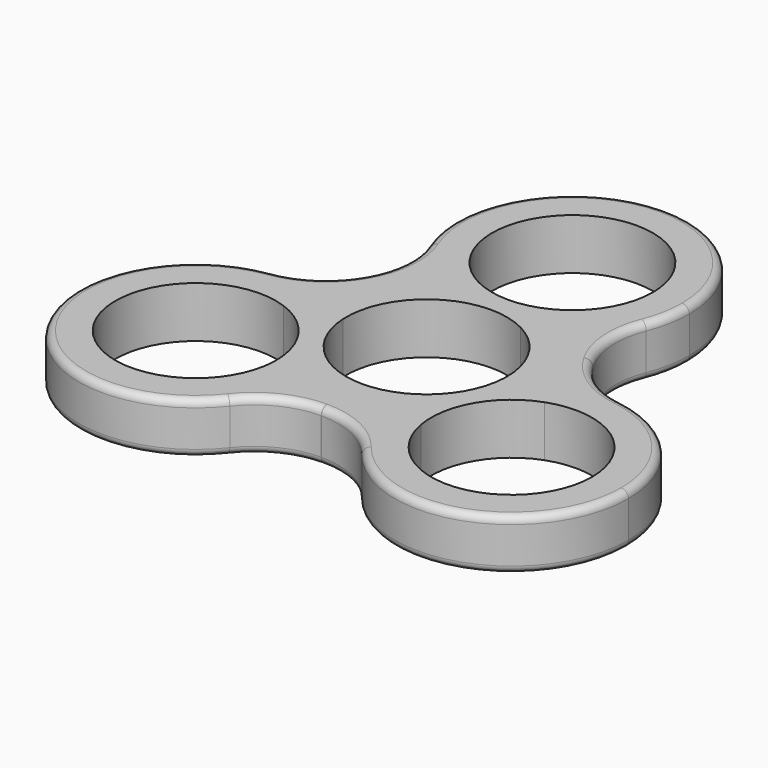
from build123d import *

# Parameters (mm, degrees)
F1_DEPTH = 7
F2_R     = 1


with BuildPart() as f1:
    # F0 (on Top) → F1 (new body)
    with BuildSketch(Plane.XY):
        with BuildLine():
            ThreePointArc((5.060494047, 9.795), (9.4165432051, 5.7340508426), (11.025, 0))
            ThreePointArc((11.025, 0), (11.0219910528, -0.2575620937), (11.0129658536, -0.5149835996))
            ThreePointArc((11.0129658536, -0.5149835996), (14.1740719643, 1.673977168), (17.7656075732, 3.0469349442))
            ThreePointArc((17.7656075732, 3.0469349442), (16.9557411525, 6.115837389), (15.6201357815, 8.9951088469))
            ThreePointArc((15.6201357815, 8.9951088469), (15.6101079032, 9.0125), (15.600060662, 9.0298799738))
            ThreePointArc((15.600060662, 9.0298799738), (13.7743411206, 11.6261838836), (11.5215268519, 13.862))
            ThreePointArc((11.5215268519, 13.862), (8.536742735, 11.4381178122), (5.060494047, 9.795))
        make_face()
        with BuildLine():
            ThreePointArc((-11.0129658536, -0.5149835996), (-9.5479300767, 5.5125), (-5.060494047, 9.795))
            ThreePointArc((-5.060494047, 9.795), (-8.536742735, 11.4381178122), (-11.5215268519, 13.862))
            ThreePointArc((-11.5215268519, 13.862), (-13.7743411206, 11.6261838836), (-15.600060662, 9.0298799738))
            ThreePointArc((-15.600060662, 9.0298799738), (-15.6101079032, 9.0125), (-15.6201357815, 8.9951088469))
            ThreePointArc((-15.6201357815, 8.9951088469), (-16.9557411525, 6.115837389), (-17.7656075732, 3.0469349442))
            ThreePointArc((-17.7656075732, 3.0469349442), (-14.1740719643, 1.673977168), (-11.0129658536, -0.5149835996))
        make_face()
        with BuildLine():
            ThreePointArc((7.1017699202, 16.567), (9.4093598037, 15.3741527599), (11.5215268519, 13.862))
            ThreePointArc((11.5215268519, 13.862), (13.4516295767, 16.2905633516), (14.8776527516, 19.0454997185))
            ThreePointArc((14.8776527516, 19.0454997185), (15.7355490903, 21.9679841973), (16.025, 25))
            ThreePointArc((16.025, 25), (-3.0320158027, 40.7355490903), (-14.8776527516, 19.0454997185))
            ThreePointArc((-14.8776527516, 19.0454997185), (-13.4516295767, 16.2905633516), (-11.5215268519, 13.862))
            ThreePointArc((-11.5215268519, 13.862), (-9.4093598037, 15.3741527599), (-7.1017699202, 16.567))
            ThreePointArc((-7.1017699202, 16.567), (-4.6504629678, 34.9961902335), (11.025, 25))
            ThreePointArc((11.025, 25), (9.9961902335, 20.3495370322), (7.1017699202, 16.567))
        make_face()
        with BuildLine():
            ThreePointArc((14.8776527516, 19.0454997185), (13.4516295767, 16.2905633516), (11.5215268519, 13.862))
            ThreePointArc((11.5215268519, 13.862), (13.7743411206, 11.6261838836), (15.600060662, 9.0298799738))
            ThreePointArc((15.600060662, 9.0298799738), (14.0855515443, 13.9545041029), (14.8776527516, 19.0454997185))
        make_face()
        with BuildLine():
            ThreePointArc((6.2440807213, -16.9089349442), (5.6373292293, -13.1120949802), (5.9524718066, -9.2800164004))
            ThreePointArc((5.9524718066, -9.2800164004), (0, -11.025), (-5.9524718066, -9.2800164004))
            ThreePointArc((-5.9524718066, -9.2800164004), (-5.7075536533, -10.8817357588), (-5.6256350946, -12.5))
            ThreePointArc((-5.6256350946, -12.5), (-5.7809996414, -14.726049322), (-6.2440807213, -16.9089349442))
            ThreePointArc((-6.2440807213, -16.9089349442), (-3.1814000319, -17.7420212726), (-0.0200751195, -18.0249888208))
            ThreePointArc((-0.0200751195, -18.0249888208), (0, -18.025), (0.0200751195, -18.0249888208))
            ThreePointArc((0.0200751195, -18.0249888208), (3.1814000319, -17.7420212726), (6.2440807213, -16.9089349442))
        make_face()
        with BuildLine():
            ThreePointArc((23.9327129598, 3.3616753723), (20.8338564928, 3.5041712599), (17.7656075732, 3.0469349442))
            ThreePointArc((17.7656075732, 3.0469349442), (17.9600348205, 1.5289781706), (18.025, 0))
            ThreePointArc((18.025, 0), (17.9933040884, -1.0684722648), (17.8983278246, -2.1331868372))
            ThreePointArc((17.8983278246, -2.1331868372), (27.982358294, -3.4744858138), (32.6756350946, -12.5))
            ThreePointArc((32.6756350946, -12.5), (22.6213111419, -23.4821861672), (10.7965579044, -14.4338131628))
            ThreePointArc((10.7965579044, -14.4338131628), (8.6097269498, -15.8358210033), (6.2440807213, -16.9089349442))
            ThreePointArc((6.2440807213, -16.9089349442), (7.3822269161, -19.7947346115), (9.0550602082, -22.4071750908))
            ThreePointArc((9.0550602082, -22.4071750908), (26.89260693, -27.643393156), (37.6756350946, -12.5))
            ThreePointArc((37.6756350946, -12.5), (33.7620124479, -2.0064227451), (23.9327129598, 3.3616753723))
        make_face()
        with BuildLine():
            ThreePointArc((15.6201357815, 8.9951088469), (16.9557411525, 6.115837389), (17.7656075732, 3.0469349442))
            ThreePointArc((17.7656075732, 3.0469349442), (20.8338564928, 3.5041712599), (23.9327129598, 3.3616753723))
            ThreePointArc((23.9327129598, 3.3616753723), (19.1277308225, 5.2211934122), (15.6201357815, 8.9951088469))
        make_face()
        with BuildLine():
            ThreePointArc((-15.600060662, 9.0298799738), (-13.7743411206, 11.6261838836), (-11.5215268519, 13.862))
            ThreePointArc((-11.5215268519, 13.862), (-13.4516295767, 16.2905633516), (-14.8776527516, 19.0454997185))
            ThreePointArc((-14.8776527516, 19.0454997185), (-14.0855515443, 13.9545041029), (-15.600060662, 9.0298799738))
        make_face()
        with BuildLine():
            ThreePointArc((9.0550602082, -22.4071750908), (7.3822269161, -19.7947346115), (6.2440807213, -16.9089349442))
            ThreePointArc((6.2440807213, -16.9089349442), (3.1814000319, -17.7420212726), (0.0200751195, -18.0249888208))
            ThreePointArc((0.0200751195, -18.0249888208), (5.0421792782, -19.1756975152), (9.0550602082, -22.4071750908))
        make_face()
        with BuildLine():
            ThreePointArc((-23.9327129598, 3.3616753723), (-20.8338564928, 3.5041712599), (-17.7656075732, 3.0469349442))
            ThreePointArc((-17.7656075732, 3.0469349442), (-16.9557411525, 6.115837389), (-15.6201357815, 8.9951088469))
            ThreePointArc((-15.6201357815, 8.9951088469), (-19.1277308225, 5.2211934122), (-23.9327129598, 3.3616753723))
        make_face()
        with BuildLine():
            ThreePointArc((-17.8983278246, -2.1331868372), (-18.0190867536, 0.4616682434), (-17.7656075732, 3.0469349442))
            ThreePointArc((-17.7656075732, 3.0469349442), (-20.8338564928, 3.5041712599), (-23.9327129598, 3.3616753723))
            ThreePointArc((-23.9327129598, 3.3616753723), (-35.5286921903, -20.5125), (-9.0550602082, -22.4071750908))
            ThreePointArc((-9.0550602082, -22.4071750908), (-7.3822269161, -19.7947346115), (-6.2440807213, -16.9089349442))
            ThreePointArc((-6.2440807213, -16.9089349442), (-8.6097269498, -15.8358210033), (-10.7965579044, -14.4338131628))
            ThreePointArc((-10.7965579044, -14.4338131628), (-31.1985651713, -18.0125), (-17.8983278246, -2.1331868372))
        make_face()
        with BuildLine():
            ThreePointArc((-0.0200751195, -18.0249888208), (-3.1814000319, -17.7420212726), (-6.2440807213, -16.9089349442))
            ThreePointArc((-6.2440807213, -16.9089349442), (-7.3822269161, -19.7947346115), (-9.0550602082, -22.4071750908))
            ThreePointArc((-9.0550602082, -22.4071750908), (-5.0421792782, -19.1756975152), (-0.0200751195, -18.0249888208))
        make_face()
        with BuildLine():
            ThreePointArc((-5.060494047, 9.795), (0, 11.025), (5.060494047, 9.795))
            ThreePointArc((5.060494047, 9.795), (8.536742735, 11.4381178122), (11.5215268519, 13.862))
            ThreePointArc((11.5215268519, 13.862), (9.4093598037, 15.3741527599), (7.1017699202, 16.567))
            ThreePointArc((7.1017699202, 16.567), (0, 13.975), (-7.1017699202, 16.567))
            ThreePointArc((-7.1017699202, 16.567), (-9.4093598037, 15.3741527599), (-11.5215268519, 13.862))
            ThreePointArc((-11.5215268519, 13.862), (-8.536742735, 11.4381178122), (-5.060494047, 9.795))
        make_face()
        with BuildLine():
            ThreePointArc((-5.9524718066, -9.2800164004), (-9.5479300767, -5.5125), (-11.0129658536, -0.5149835996))
            ThreePointArc((-11.0129658536, -0.5149835996), (-14.1740719643, 1.673977168), (-17.7656075732, 3.0469349442))
            ThreePointArc((-17.7656075732, 3.0469349442), (-18.0190867536, 0.4616682434), (-17.8983278246, -2.1331868372))
            ThreePointArc((-17.8983278246, -2.1331868372), (-12.6251209084, -6.1682768006), (-10.6256350946, -12.5))
            ThreePointArc((-10.6256350946, -12.5), (-10.6684489274, -13.4706760473), (-10.7965579044, -14.4338131628))
            ThreePointArc((-10.7965579044, -14.4338131628), (-8.6097269498, -15.8358210033), (-6.2440807213, -16.9089349442))
            ThreePointArc((-6.2440807213, -16.9089349442), (-5.7809996414, -14.726049322), (-5.6256350946, -12.5))
            ThreePointArc((-5.6256350946, -12.5), (-5.7075536533, -10.8817357588), (-5.9524718066, -9.2800164004))
        make_face()
        with BuildLine():
            ThreePointArc((17.7656075732, 3.0469349442), (14.1740719643, 1.673977168), (11.0129658536, -0.5149835996))
            ThreePointArc((11.0129658536, -0.5149835996), (9.5479300767, -5.5125), (5.9524718066, -9.2800164004))
            ThreePointArc((5.9524718066, -9.2800164004), (5.6373292293, -13.1120949802), (6.2440807213, -16.9089349442))
            ThreePointArc((6.2440807213, -16.9089349442), (8.6097269498, -15.8358210033), (10.7965579044, -14.4338131628))
            ThreePointArc((10.7965579044, -14.4338131628), (12.1027050179, -6.9875), (17.8983278246, -2.1331868372))
            ThreePointArc((17.8983278246, -2.1331868372), (17.9933040884, -1.0684722648), (18.025, 0))
            ThreePointArc((18.025, 0), (17.9600348205, 1.5289781706), (17.7656075732, 3.0469349442))
        make_face()
    extrude(amount=F1_DEPTH)

    # F2
    f2_edges = [f1.edges().sort_by_distance(p)[0] for p in [
        (14.877653, 19.0455, 3.5),
        (-14.877653, 19.0455, 3.5),
        (0, 41.025, 0),
        (0, 41.025, 7),
        (-15.600061, 9.02988, 3.5),
        (-14.085552, 13.954504, 0),
        (-14.085552, 13.954504, 7),
        (-15.620136, 8.995109, 3.5),
        (-23.932713, 3.361675, 3.5),
        (-19.127731, 5.221193, 0),
        (-19.127731, 5.221193, 7),
        (-9.05506, -22.407175, 3.5),
        (-35.528692, -20.5125, 0),
        (-35.528692, -20.5125, 7),
        (0.020075, -18.024989, 3.5),
        (9.05506, -22.407175, 3.5),
        (5.042179, -19.175698, 0),
        (5.042179, -19.175698, 7),
    ]]
    fillet(f2_edges, radius=F2_R)


solid = f1.part
